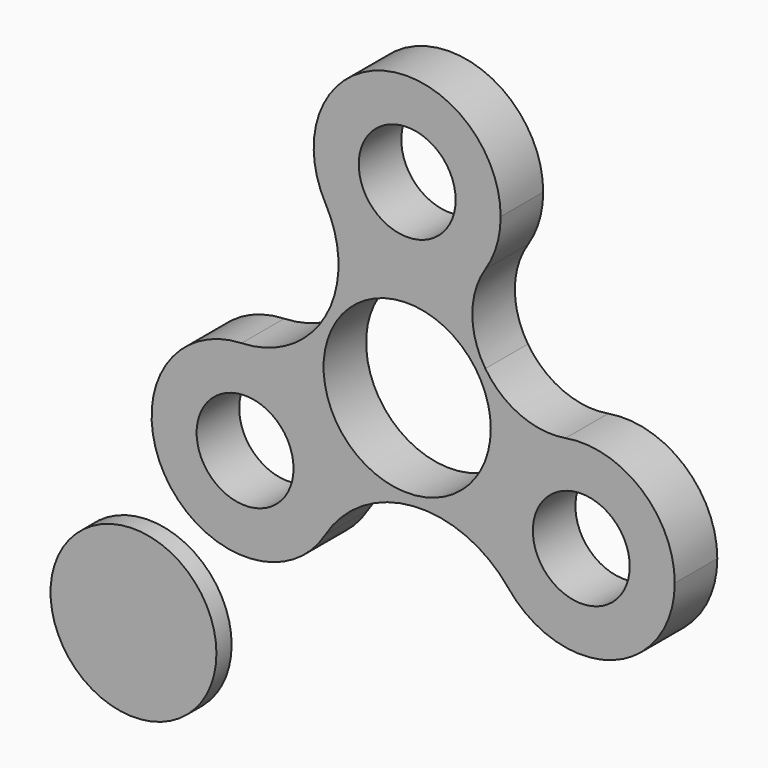
from build123d import *

# Parameters (mm, degrees)
F0_R     = 6.375
F0_R_2   = 11
F1_DEPTH = 7
F2_R     = 10.915
F2_R_2   = 4.5
F3_DEPTH = 2.5


# Not quite as in the source:
# - a feature names something its author has since deleted; it is built from what else it names
# - the program builds the solid bodies; features that only make, move or delete a surface that nothing else refers to are left out


with BuildPart() as f1:
    # F0 (on Front) → F1 (new body)
    with BuildSketch(Plane.XZ):
        with BuildLine():
            ThreePointArc((10.2913244925, 18.2636330126), (11.7871389925, 21.4852661024), (12.3, 25))
            ThreePointArc((12.3, 25), (-3.1089572961, 36.9006043767), (-10.7283552083, 18.983988487))
            ThreePointArc((-10.7283552083, 18.983988487), (-0.4212801491, 12.7072166278), (10.2913244925, 18.2636330126))
        make_face()
        with Locations((0, 25)):
            Circle(F0_R, mode=Mode.SUBTRACT)
        with BuildLine():
            ThreePointArc((10.2913244925, 18.2636330126), (-0.4212801491, 12.7072166278), (-10.7283552083, 18.983988487))
            ThreePointArc((-10.7283552083, 18.983988487), (-9.0344544049, 12.4999999397), (-10.7283552673, 6.0160114077))
            ThreePointArc((-10.7283552673, 6.0160114077), (-0.4212802335, 12.2927833693), (10.2913244661, 6.7363670278))
            ThreePointArc((10.2913244661, 6.7363670278), (8.5727024982, 12.5000000241), (10.2913244925, 18.2636330126))
        make_face()
        with BuildLine():
            ThreePointArc((10.2913244661, 6.7363670278), (-0.4212802335, 12.2927833693), (-10.7283552673, 6.0160114077))
            ThreePointArc((-10.7283552673, 6.0160114077), (-10.3942134043, -6.576498134), (0.8420661962, -12.2711419404))
            ThreePointArc((0.8420661962, -12.2711419404), (8.9902006155, -8.3944203429), (12.3, 0))
            ThreePointArc((12.3, 0), (11.7871389856, 3.5147339207), (10.2913244661, 6.7363670278))
        make_face()
        Circle(F0_R_2, mode=Mode.SUBTRACT)
        with BuildLine():
            ThreePointArc((0.8420661962, -12.2711419404), (-10.3942134043, -6.576498134), (-10.7283552673, 6.0160114077))
            ThreePointArc((-10.7283552673, 6.0160114077), (-15.3771779341, 1.1890192116), (-21.7929065021, -0.7474292877))
            ThreePointArc((-21.7929065021, -0.7474292877), (-12.7981553136, -4.1793542246), (-9.0305269511, -13.0387353677))
            ThreePointArc((-9.0305269511, -13.0387353677), (-9.4793966749, -16.3312588946), (-10.7932442154, -19.3834711816))
            ThreePointArc((-10.7932442154, -19.3834711816), (-5.8461277368, -14.4031615344), (0.8420661962, -12.2711419404))
        make_face()
        with BuildLine():
            ThreePointArc((20.8556822396, 2.1241866562), (14.8858646149, 2.8552166619), (10.2913244661, 6.7363670278))
            ThreePointArc((10.2913244661, 6.7363670278), (11.7871389856, 3.5147339207), (12.3, 0))
            ThreePointArc((12.3, 0), (8.9902006155, -8.3944203429), (0.8420661962, -12.2711419404))
            ThreePointArc((0.8420661962, -12.2711419404), (7.7588005924, -13.4695690785), (13.3398545128, -17.7274182361))
            ThreePointArc((13.3398545128, -17.7274182361), (11.4084974744, -5.6476549278), (20.8556822396, 2.1241866562))
        make_face()
        with BuildLine():
            ThreePointArc((-9.0305269511, -13.0387353677), (-12.7981553136, -4.1793542246), (-21.7929065021, -0.7474292877))
            ThreePointArc((-21.7929065021, -0.7474292877), (-31.9230447308, -19.2908203869), (-10.7932442154, -19.3834711816))
            ThreePointArc((-10.7932442154, -19.3834711816), (-9.4793966749, -16.3312588946), (-9.0305269511, -13.0387353677))
        make_face()
        with Locations((-21.3305269511, -13.0387353677)):
            Circle(F0_R, mode=Mode.SUBTRACT)
        with BuildLine():
            ThreePointArc((35.2116724729, -10.0027628432), (30.8489679862, -0.606522109), (20.8556822396, 2.1241866562))
            ThreePointArc((20.8556822396, 2.1241866562), (11.4084974744, -5.6476549278), (13.3398545128, -17.7274182361))
            ThreePointArc((13.3398545128, -17.7274182361), (27.0078071808, -21.6006799171), (35.2116724729, -10.0027628432))
        make_face()
        with Locations((22.9116724729, -10.0027628432)):
            Circle(F0_R, mode=Mode.SUBTRACT)
    extrude(amount=F1_DEPTH)


with BuildPart() as f3:
    # F2 (on Front) → F3 (new body)
    with BuildSketch(Plane.XZ):
        with Locations((-39.6157391369, -40.7749339938)):
            Circle(F2_R)
        with Locations((-39.6157391369, -40.7749339938)):
            Circle(F2_R_2, mode=Mode.SUBTRACT)
        with Locations((-39.6157391369, -40.7749339938)):
            Circle(F2_R_2)
    extrude(amount=F3_DEPTH)


solid = Compound([f1.part, f3.part])
